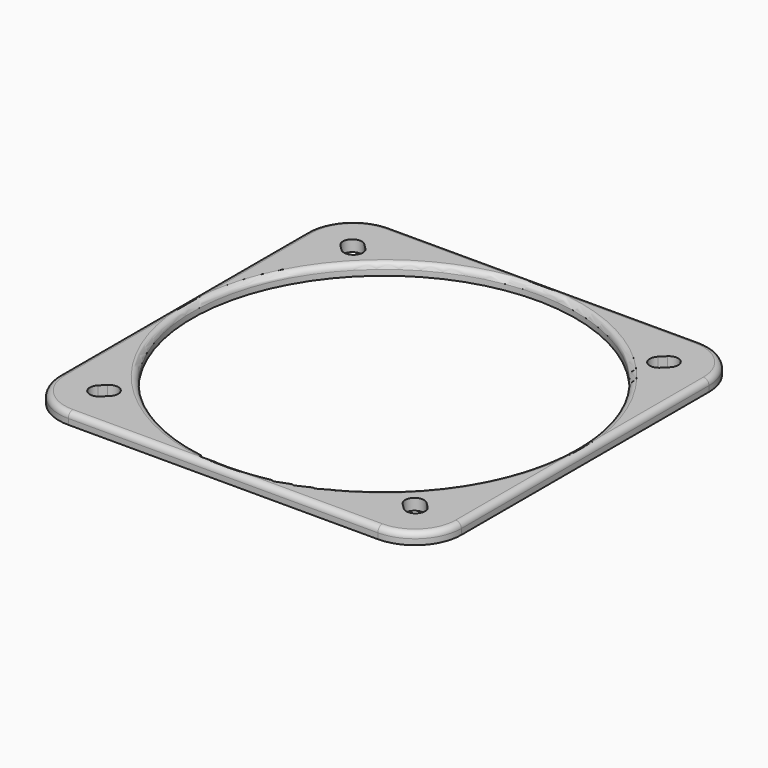
from build123d import *

# Parameters (mm, degrees)
F0_R         = 51
F1_DEPTH     = 3
F2_T1_DEPTH  = 82.316462509
F2_T3_DEPTH  = 82.316462509
F2_T6_ANGLE  = 90
F2_T8_ANGLE  = 90
F2_T10_ANGLE = 90
F2_T12_ANGLE = 90


# Not quite as in the source:
# - a fillet or chamfer that OpenCascade refuses, or shapes differently, is made with other operations: its cross-section is extruded or revolved along the edge and cut away or added


with BuildPart() as f1:
    # F0 (on Top) → F1 (new body)
    with BuildSketch(Plane.XY):
        with BuildLine():
            Line((41.1582312545, 53.5), (-41.1582312545, 53.5))
            ThreePointArc((-41.1582312545, 53.5), (-49.8851796263, 49.8851796263), (-53.5, 41.1582312545))
            Line((-53.5, 41.1582312545), (-53.5, -41.1582312545))
            ThreePointArc((-53.5, -41.1582312545), (-49.8851796263, -49.8851796263), (-41.1582312545, -53.5))
            Line((-41.1582312545, -53.5), (41.1582312545, -53.5))
            ThreePointArc((41.1582312545, -53.5), (49.8851796263, -49.8851796263), (53.5, -41.1582312545))
            Line((53.5, -41.1582312545), (53.5, 41.1582312545))
            ThreePointArc((53.5, 41.1582312545), (49.8851796263, 49.8851796263), (41.1582312545, 53.5))
        make_face()
        with BuildLine():
            ThreePointArc((-40.3050865276, -43.8406204336), (-43.8406204336, -43.8406204336), (-43.8406204336, -40.3050865276))
            Line((-43.8406204336, -40.3050865276), (-42.4264068712, -38.8908729653))
            ThreePointArc((-42.4264068712, -38.8908729653), (-38.8908729653, -38.8908729653), (-38.8908729653, -42.4264068712))
            Line((-38.8908729653, -42.4264068712), (-40.3050865276, -43.8406204336))
        make_face(mode=Mode.SUBTRACT)
        Circle(F0_R, mode=Mode.SUBTRACT)
        with BuildLine():
            ThreePointArc((43.8406204336, -40.3050865276), (43.8406204336, -43.8406204336), (40.3050865276, -43.8406204336))
            Line((40.3050865276, -43.8406204336), (38.8908729653, -42.4264068712))
            ThreePointArc((38.8908729653, -42.4264068712), (38.8908729653, -38.8908729653), (42.4264068712, -38.8908729653))
            Line((42.4264068712, -38.8908729653), (43.8406204336, -40.3050865276))
        make_face(mode=Mode.SUBTRACT)
        with BuildLine():
            ThreePointArc((-43.8406204336, 40.3050865276), (-43.8406204336, 43.8406204336), (-40.3050865276, 43.8406204336))
            Line((-40.3050865276, 43.8406204336), (-38.8908729653, 42.4264068712))
            ThreePointArc((-38.8908729653, 42.4264068712), (-38.8908729653, 38.8908729653), (-42.4264068712, 38.8908729653))
            Line((-42.4264068712, 38.8908729653), (-43.8406204336, 40.3050865276))
        make_face(mode=Mode.SUBTRACT)
        with BuildLine():
            ThreePointArc((40.3050865276, 43.8406204336), (43.8406204336, 43.8406204336), (43.8406204336, 40.3050865276))
            Line((43.8406204336, 40.3050865276), (42.4264068712, 38.8908729653))
            ThreePointArc((42.4264068712, 38.8908729653), (38.8908729653, 38.8908729653), (38.8908729653, 42.4264068712))
            Line((38.8908729653, 42.4264068712), (40.3050865276, 43.8406204336))
        make_face(mode=Mode.SUBTRACT)
    extrude(amount=F1_DEPTH)

    # F2: fillet of radius 1.5 on 8 edges, made by hand

    # F2_s2 → F2_t1 (cut)
    with BuildSketch(Plane.XZ.offset(-41.1582312545)):
        with BuildLine():
            ThreePointArc((-53.5, 1.5), (-53.0606601718, 2.5606601718), (-52, 3))
            Line((-52, 3), (-53.5, 3))
            Line((-53.5, 3), (-53.5, 1.5))
        make_face()
        with BuildLine():
            ThreePointArc((53.5, 1.5), (53.0606601718, 2.5606601718), (52, 3))
            Line((52, 3), (53.5, 3))
            Line((53.5, 3), (53.5, 1.5))
        make_face()
    extrude(amount=F2_T1_DEPTH, mode=Mode.SUBTRACT)

    # F2_s4 → F2_t3 (cut)
    with BuildSketch(Plane.YZ.offset(-41.1582312545)):
        with BuildLine():
            ThreePointArc((53.5, 1.5), (53.0606601718, 2.5606601718), (52, 3))
            Line((52, 3), (53.5, 3))
            Line((53.5, 3), (53.5, 1.5))
        make_face()
        with BuildLine():
            ThreePointArc((-53.5, 1.5), (-53.0606601718, 2.5606601718), (-52, 3))
            Line((-52, 3), (-53.5, 3))
            Line((-53.5, 3), (-53.5, 1.5))
        make_face()
    extrude(amount=F2_T3_DEPTH, mode=Mode.SUBTRACT)

    # F2_s5 → F2_t6 (revolve, cut)
    with BuildSketch(Plane.YZ.offset(-41.1582312545)):
        with BuildLine():
            ThreePointArc((53.5, 1.5), (53.0606601718, 2.5606601718), (52, 3))
            Line((52, 3), (53.5, 3))
            Line((53.5, 3), (53.5, 1.5))
        make_face()
    revolve(axis=Axis((-41.1582312545, 41.1582312545, 3), (0, 0, 1)), revolution_arc=F2_T6_ANGLE, mode=Mode.SUBTRACT)

    # F2_s7 → F2_t8 (revolve, cut)
    with BuildSketch(Plane.XZ.offset(-41.1582312545)):
        with BuildLine():
            ThreePointArc((53.5, 1.5), (53.0606601718, 2.5606601718), (52, 3))
            Line((52, 3), (53.5, 3))
            Line((53.5, 3), (53.5, 1.5))
        make_face()
    revolve(axis=Axis((41.1582312545, 41.1582312545, 3), (0, 0, 1)), revolution_arc=F2_T8_ANGLE, mode=Mode.SUBTRACT)

    # F2_s9 → F2_t10 (revolve, cut)
    with BuildSketch(Plane.XZ.offset(41.1582312545)):
        with BuildLine():
            ThreePointArc((-53.5, 1.5), (-53.0606601718, 2.5606601718), (-52, 3))
            Line((-52, 3), (-53.5, 3))
            Line((-53.5, 3), (-53.5, 1.5))
        make_face()
    revolve(axis=Axis((-41.1582312545, -41.1582312545, 3), (0, 0, 1)), revolution_arc=F2_T10_ANGLE, mode=Mode.SUBTRACT)

    # F2_s11 → F2_t12 (revolve, cut)
    with BuildSketch(Plane.YZ.offset(41.1582312545)):
        with BuildLine():
            ThreePointArc((-53.5, 1.5), (-53.0606601718, 2.5606601718), (-52, 3))
            Line((-52, 3), (-53.5, 3))
            Line((-53.5, 3), (-53.5, 1.5))
        make_face()
    revolve(axis=Axis((41.1582312545, -41.1582312545, 3), (0, 0, 1)), revolution_arc=F2_T12_ANGLE, mode=Mode.SUBTRACT)

    # F2_s13 → F2_t14 (revolve, cut)
    with BuildSketch(Plane.XZ):
        with BuildLine():
            ThreePointArc((51, 1.5), (51.4393398282, 2.5606601718), (52.5, 3))
            Line((52.5, 3), (51, 3))
            Line((51, 3), (51, 1.5))
        make_face()
    revolve(axis=Axis((0, 0, 3), (0, 0, 1)), mode=Mode.SUBTRACT)


solid = f1.part
